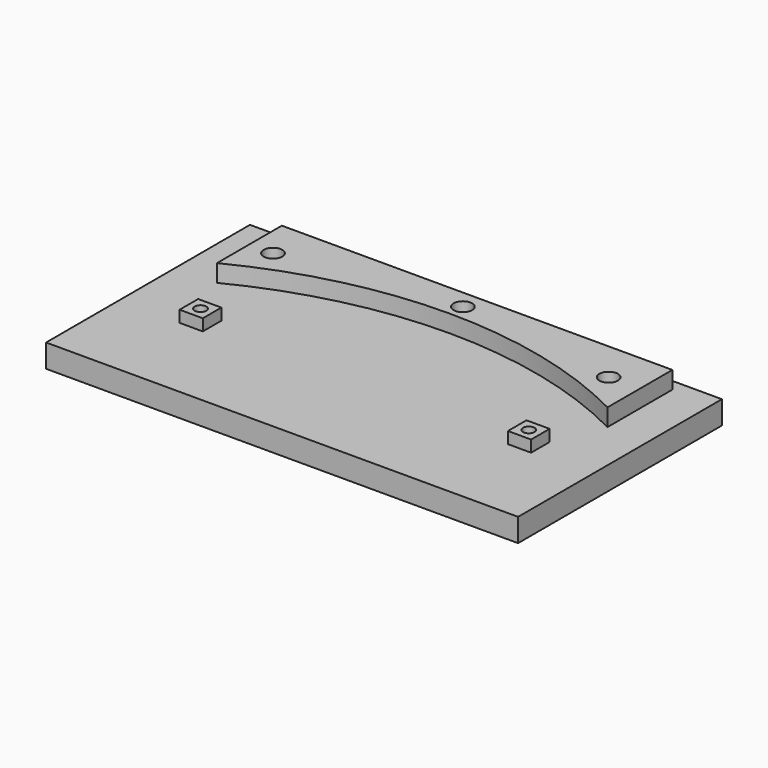
from build123d import *

# Parameters (mm, degrees)
F0_R     = 4
F1_DEPTH = 7.5
F0_R_2   = 2.5
F2_DEPTH = 5
F0_W     = 203.6497449993
F0_H     = 109.9428115989
F4_DEPTH = 10


# Not quite as in the source:
# - the program builds the solid bodies; features that only make, move or delete a surface that nothing else refers to are left out


with BuildPart() as f1:
    # F0 (on Top) → F1 (new body)
    with BuildSketch(Plane.XY):
        with BuildLine():
            Line((84.4433900163, 14.9714057995), (84.4433900163, 49.9714057995))
            Line((84.4433900163, 49.9714057995), (-84.0557436719, 49.9714057995))
            Line((-84.0557436719, 49.9714057995), (-84.0557436719, 14.9714057995))
            ThreePointArc((-84.0557436719, 14.9714057995), (0.1938231722, 35.2128277571), (84.4433900163, 14.9714057995))
        make_face()
        with Locations((-73.8124497916, 32.3899931005)):
            Circle(F0_R, mode=Mode.SUBTRACT)
        with Locations((0.5230791285, 41.8811105192)):
            Circle(F0_R, mode=Mode.SUBTRACT)
        with Locations((71.0174008963, 32.3899931005)):
            Circle(F0_R, mode=Mode.SUBTRACT)
    extrude(amount=F1_DEPTH)


with BuildPart() as f2:
    # F0 (on Top) → F2 (new body)
    with BuildSketch(Plane.XY):
        Polygon((-65.6322131381, -15.68778418), (-65.6322131381, -8.2608617701), (-65.6322131381, -5.68778418), (-75.6322131381, -5.68778418), (-75.6322131381, -15.68778418), align=None)
        with Locations((-70.6322131381, -10.68778418)):
            Circle(F0_R_2, mode=Mode.SUBTRACT)
    extrude(amount=F2_DEPTH)


with BuildPart() as f2b:
    # F0 (on Top) → F2, piece 2 (new body)
    with BuildSketch(Plane.XY):
        Polygon((66.0198594824, -5.68778418), (66.0198594824, -8.2608617701), (66.0198594824, -15.68778418), (76.0198594824, -15.68778418), (76.0198594824, -5.68778418), align=None)
        with Locations((71.0198594824, -10.68778418)):
            Circle(F0_R_2, mode=Mode.SUBTRACT)
    extrude(amount=F2_DEPTH)


with BuildPart() as f4:
    # F0 (on Top) → F4 (new body)
    with BuildSketch(Plane.XY):
        Rectangle(F0_W, F0_H)
        Polygon((-65.6322131381, -5.68778418), (-65.6322131381, -8.2608617701), (-65.6322131381, -15.68778418), (-75.6322131381, -15.68778418), (-75.6322131381, -5.68778418), align=None, mode=Mode.SUBTRACT)
        Polygon((66.0198594824, -15.68778418), (66.0198594824, -8.2608617701), (66.0198594824, -5.68778418), (76.0198594824, -5.68778418), (76.0198594824, -15.68778418), align=None, mode=Mode.SUBTRACT)
        with BuildLine():
            Line((-84.0557436719, 49.9714057995), (84.4433900163, 49.9714057995))
            Line((84.4433900163, 49.9714057995), (84.4433900163, 14.9714057995))
            ThreePointArc((84.4433900163, 14.9714057995), (0.1938231722, 35.2128277571), (-84.0557436719, 14.9714057995))
            Line((-84.0557436719, 14.9714057995), (-84.0557436719, 49.9714057995))
        make_face(mode=Mode.SUBTRACT)
    extrude(amount=-F4_DEPTH)


solid = Compound([f1.part, f2.part, f2b.part, f4.part])
